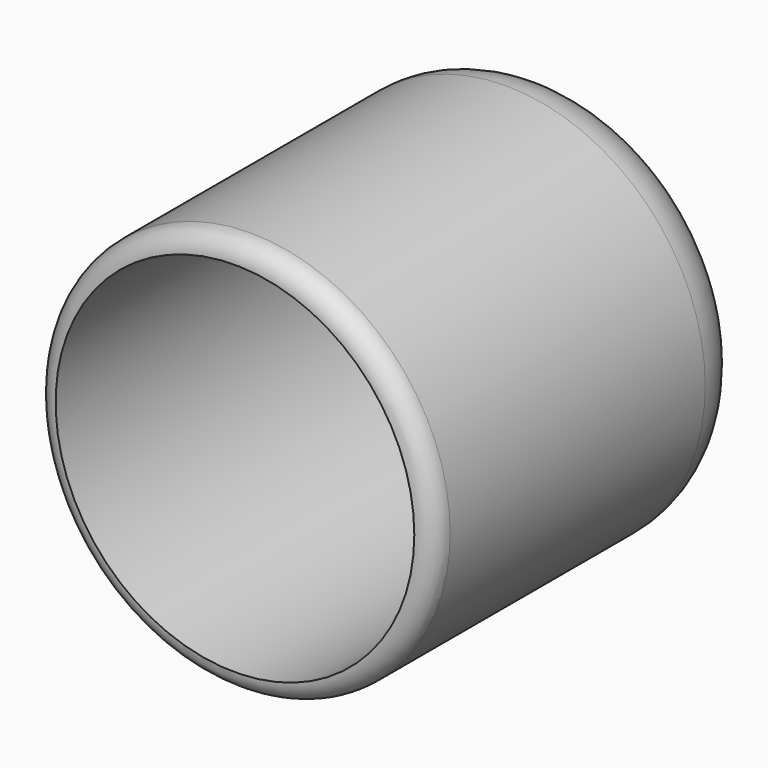
from build123d import *

# Parameters (mm, degrees)
F0_R     = 50.8
F1_DEPTH = 101.6
F2_T     = -5.08
F3_R     = 15.24
F4_R     = 5.07999


# Not quite as in the source:
# - a fillet or chamfer is up to 0.001 mm smaller than in the source, because OpenCascade refuses the exact size


with BuildPart() as f1:
    # F0 (on Front) → F1 (new body)
    with BuildSketch(Plane.XZ):
        Circle(F0_R)
    extrude(amount=F1_DEPTH)

    # F2
    f2_openings = [f1.faces().sort_by_distance(p)[0] for p in [
        (0, -101.6, 0),
    ]]
    offset(amount=F2_T, openings=f2_openings)

    # F3
    f3_edges = [f1.edges().sort_by_distance(p)[0] for p in [
        (-50.8, 0, 0),
    ]]
    fillet(f3_edges, radius=F3_R)

    # F4 (radius 5.08 in the source; OpenCascade refuses exactly that, so slightly less here)
    f4_edges = [f1.edges().sort_by_distance(p)[0] for p in [
        (-50.8, -101.6, 0),
    ]]
    fillet(f4_edges, radius=F4_R)


solid = f1.part
